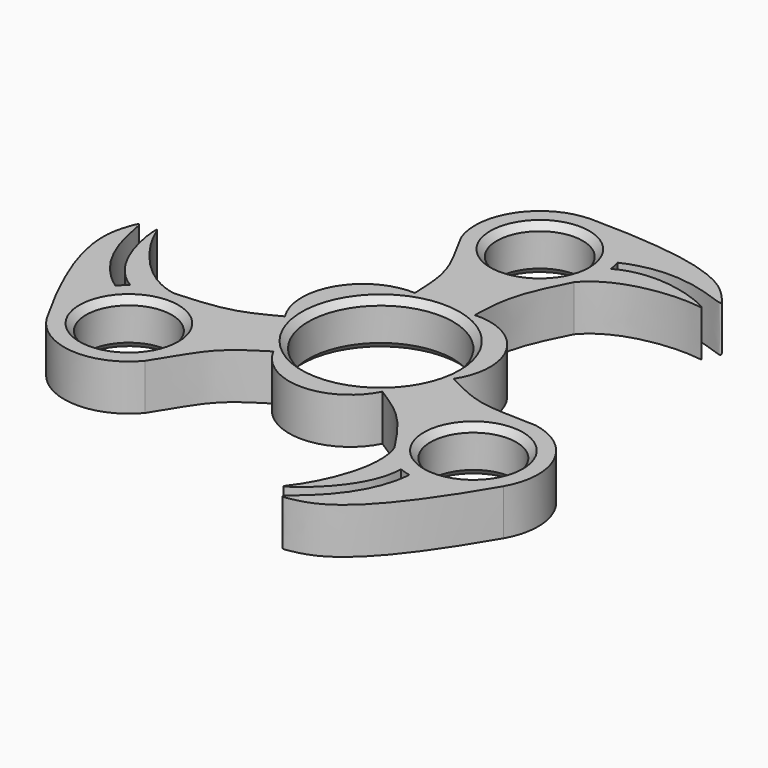
from build123d import *

# Parameters (mm, degrees)
F0_R     = 6.55
F0_R_2   = 11.05
F1_DEPTH = 7
F2_SIZE  = 1


# Not quite as in the source:
# - ends of sketch curves that miss each other by under 0.0002 mm in the source are joined


with BuildPart() as f1:
    # F0 (on Top) → F1 (new body)
    with BuildSketch(Plane.XY):
        with BuildLine():
            ThreePointArc((0, 40.1977714043), (-8.0681283552, 36.0092836242), (-9.2850536357, 27.0005535305))
            add(Edge.make_bspline(
                [(-9.2850536357, 27.0005535305), (-7.6485537074, 23.76762968), (-4.7701185707, 19.4412735204), (-4.6697456794, 14.4884170356), (-4.5648748072, 12.2255101831)],
                knots=[0, 0, 0, 0, 0.5344080552, 1, 1, 1, 1], degree=3))
            ThreePointArc((-4.5648748072, 12.2255101831), (-13.112130235, 7.5702762234), (-12.8700869391, -2.1594819242))
            add(Edge.make_bspline(
                [(-26.9423555096, -5.7646466266), (-24.1168902387, -5.6160652927), (-18.509620442, -5.2218898403), (-14.7902779868, -3.1525456922), (-12.8700869391, -2.1594819242)],
                knots=[0.1344901828, 0.1344901828, 0.1344901828, 0.1344901828, 0.5556800273, 1, 1, 1, 1], degree=3))
            add(Edge.make_bspline(
                [(-32.3070856345, -7.3652547262), (-38.1561546686, -3.8908306821), (-39.2425077068, 7.9341737596), (-37.973119311, 3.3638390897), (-32.4811016658, -4.8031550223), (-26.9423555096, -5.7646466266)],
                knots=[0, 0, 0, 0, 0.4276612867, 0.5658731858, 1, 1, 1, 1], degree=3))
            ThreePointArc((-32.3070856345, -7.3652547262), (-32.9876607035, -7.9431032983), (-33.6132053721, -8.5801160647))
            add(Edge.make_bspline(
                [(-34.8122912116, -20.0988857021), (-44.0385765115, -3.9019687515), (-42.749663868, 2.1665983757), (-40.6223387742, 7.8779194346), (-40.8804383129, -3.4972060171), (-33.6132053721, -8.5801160647)],
                knots=[0, 0, 0, 0, 0.4894381035, 0.610016492, 1, 1, 1, 1], degree=3))
            ThreePointArc((-34.8122912116, -20.0988857021), (-27.150890213, -24.9918459287), (-18.7406384558, -21.5413690893))
            add(Edge.make_bspline(
                [(-18.7406384558, -21.5413690893), (-16.7590942369, -18.5076566528), (-14.4515774653, -13.8516806215), (-10.2124643737, -11.2883269054), (-8.3051649892, -10.0660526397)],
                knots=[0, 0, 0, 0, 0.5344080552, 1, 1, 1, 1], degree=3))
            ThreePointArc((-8.3051649892, -10.0660526397), (1.35944e-05, -15.1405759929), (8.3052096749, -10.0660812761))
            add(Edge.make_bspline(
                [(18.4635081773, -20.4504409958), (16.9221003321, -18.0778069606), (13.7770994784, -13.4188565971), (10.1253236494, -11.2324836195), (8.3052096749, -10.0660812761)],
                knots=[0.1344901828, 0.1344901828, 0.1344901828, 0.1344901828, 0.5556800273, 1, 1, 1, 1], degree=3))
            add(Edge.make_bspline(
                [(22.5320405154, -24.2961295186), (22.4476355468, -31.0987839127), (12.7500578195, -37.9520954621), (16.0733895496, -34.5676055291), (20.4002051005, -25.7278816743), (18.4635081773, -20.4504409958)],
                knots=[0, 0, 0, 0, 0.4276612867, 0.5658731858, 1, 1, 1, 1], degree=3))
            ThreePointArc((22.5320405154, -24.2961295186), (23.3727595929, -24.5966005315), (24.2372011654, -24.8198317225))
            add(Edge.make_bspline(
                [(34.8122912116, -20.0988857021), (25.3984923193, -36.1875416297), (19.4985027008, -38.1055941008), (13.4886910278, -39.1189370569), (23.4688884096, -33.6548950882), (24.2372011654, -24.8198317225)],
                knots=[0, 0, 0, 0, 0.4894381035, 0.610016492, 1, 1, 1, 1], degree=3))
            ThreePointArc((34.8122912116, -20.0988857021), (35.2190185683, -11.0174376955), (28.0256920915, -5.4591844412))
            add(Edge.make_bspline(
                [(28.0256920915, -5.4591844412), (24.4076479443, -5.2599730272), (19.221696036, -5.5895928989), (14.8822100532, -3.2000901302), (12.8700397964, -2.1594575434)],
                knots=[0, 0, 0, 0, 0.5344080552, 1, 1, 1, 1], degree=3))
            ThreePointArc((12.8700397964, -2.1594575434), (13.1121166406, 7.5702997695), (4.5648772642, 12.2255632002))
            add(Edge.make_bspline(
                [(8.4788473323, 26.2150876224), (7.1947899065, 23.6938722533), (4.7325209636, 18.6407464373), (4.6649543374, 14.3850293117), (4.5648772642, 12.2255632002)],
                knots=[0.1344901828, 0.1344901828, 0.1344901828, 0.1344901828, 0.5556800273, 1, 1, 1, 1], degree=3))
            add(Edge.make_bspline(
                [(9.775045119, 31.6613842448), (15.7085191218, 34.9896145947), (26.4924498873, 30.0179217024), (21.8997297614, 31.2037664394), (12.0808965652, 30.5310366966), (8.4788473323, 26.2150876224)],
                knots=[0, 0, 0, 0, 0.4276612867, 0.5658731858, 1, 1, 1, 1], degree=3))
            ThreePointArc((9.775045119, 31.6613842448), (9.6149011106, 32.5397038298), (9.3760042066, 33.3999477872))
            add(Edge.make_bspline(
                [(0, 40.1977714043), (18.6400841922, 40.0895103812), (23.2511611671, 35.9389957251), (27.1336477464, 31.2410176223), (17.4115499033, 37.1521011054), (9.3760042066, 33.3999477872)],
                knots=[0, 0, 0, 0, 0.4894381035, 0.610016492, 1, 1, 1, 1], degree=3))
        make_face()
        with Locations((-26.2690269878, -15.1664298028)):
            Circle(F0_R, mode=Mode.SUBTRACT)
        Circle(F0_R_2, mode=Mode.SUBTRACT)
        with Locations((26.2690269878, -15.1664298028)):
            Circle(F0_R, mode=Mode.SUBTRACT)
        with Locations((0, 30.3328596056)):
            Circle(F0_R, mode=Mode.SUBTRACT)
    extrude(amount=F1_DEPTH)

    # F2
    f2_edges = [f1.edges().sort_by_distance(p)[0] for p in [
        (-11.05, 0, 0),
        (19.719027, -15.16643, 0),
        (-6.55, 30.33286, 0),
        (-32.819027, -15.16643, 0),
        (-6.55, 30.33286, 7),
        (-32.819027, -15.16643, 7),
        (11.05, 0, 3.5),
        (-11.05, 0, 7),
        (19.719027, -15.16643, 7),
    ]]
    chamfer(f2_edges, length=F2_SIZE)


solid = f1.part
